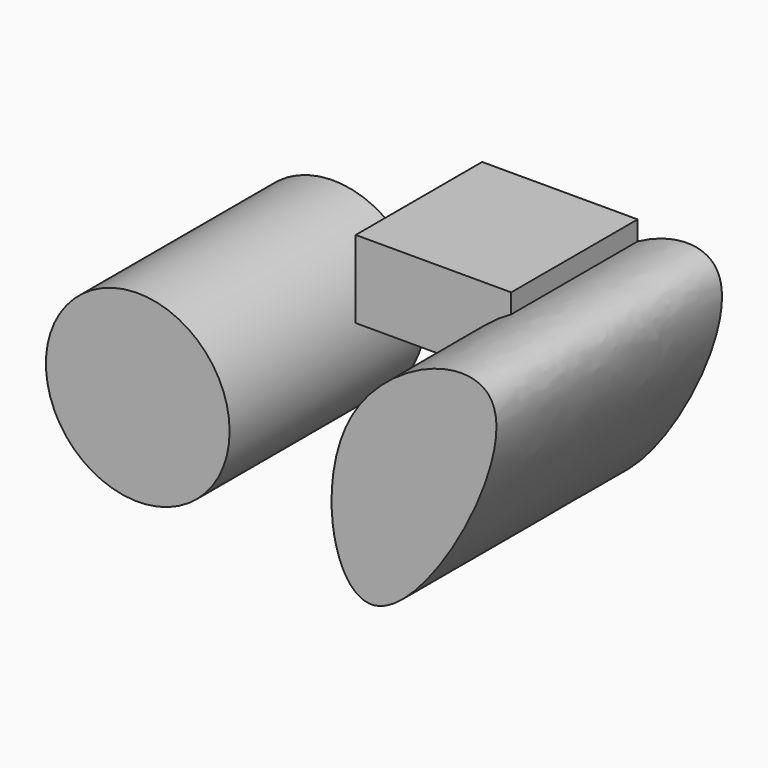
from build123d import *

# Parameters (mm, degrees)
F0_W     = 55.4656796157
F0_H     = 27.6757963002
F1_DEPTH = 56.388
F3_DEPTH = 100.584
F4_R     = 32.7676848389
F5_DEPTH = 87.122


# Not quite as in the source:
# - the program builds the solid bodies; features that only make, move or delete a surface that nothing else refers to are left out


with BuildPart() as f1:
    # F0 (on Front) → F1 (new body)
    with BuildSketch(Plane.XZ):
        with Locations((-86.2072575837, 13.8378981501)):
            Rectangle(F0_W, F0_H)
    extrude(amount=F1_DEPTH)

    # F2 (on Front) → F3 (join)
    with BuildSketch(Plane.XZ):
        with BuildLine():
            add(Edge.make_bspline(
                [(-79.9281299114, 0), (-67.0930481433, 22.5193468072), (3.5177028216, 48.0479908411), (-79.4689797754, -102.0854924294), (-93.1701175455, -23.2332693579), (-79.9281299114, 0)],
                knots=[0, 0, 0, 0, 0.3023771538, 0.6880366948, 1, 1, 1, 1], degree=3))
        make_face()
    extrude(amount=F3_DEPTH)


with BuildPart() as f5:
    # F4 (on Front) → F5 (new body)
    with BuildSketch(Plane.XZ):
        with Locations((-167.1092659235, -28.1554553658)):
            Circle(F4_R)
    extrude(amount=F5_DEPTH)


solid = Compound([f1.part, f5.part])
